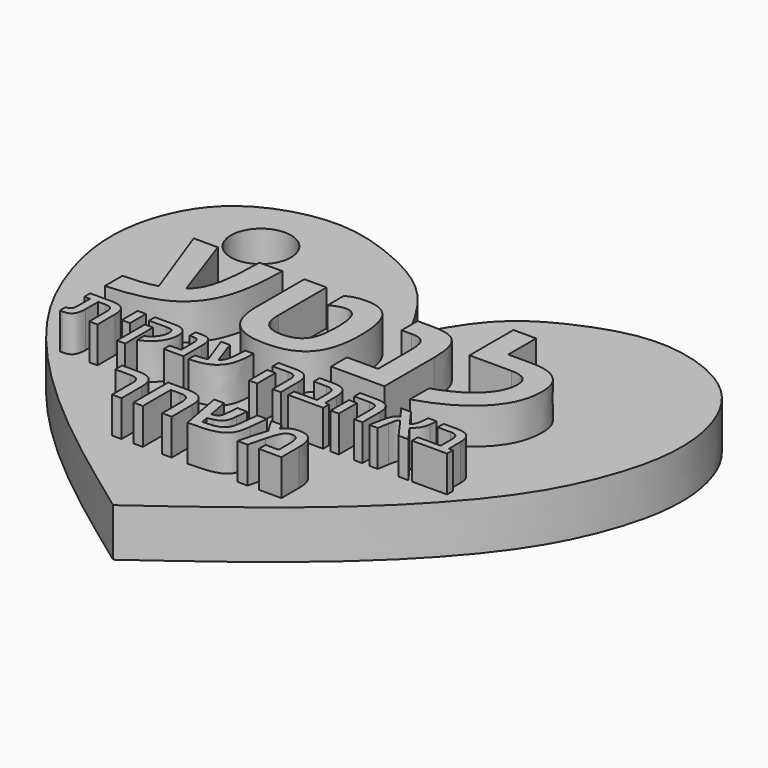
from build123d import *

# Parameters (mm, degrees)
F0_R           = 2.5
F1_DEPTH       = 4
F2_TEXT_SIZE   = 14.0530625626
F2_TEXT_SIZE_2 = 5.158657875
F2_TEXT_SIZE_3 = 5.963041874
F3_DEPTH       = 3


# Not quite as in the source:
# - Text() gives the source's letters only with a copy of the font that has no kerning and outlines rounded to 1/6400 em; it was checked with that copy


with BuildPart() as f1:
    # F0 (on Top) → F1 (new body)
    with BuildSketch(Plane.XY):
        with BuildLine():
            add(Edge.make_bspline(
                [(0, 5.3673270297), (1.0032991044, 7.2393540908), (2.9764144717, 10.9419577985), (8.4632974418, 13.8018463575), (14.0117512611, 15.2986169526), (21.7279250343, 12.71718942), (24.424666159, 4.9653958185), (22.8768308197, -1.7442714777), (20.2212687569, -7.2813165065), (15.2654507926, -13.1843862096), (8.641162767, -19.0683200173), (2.9548744589, -23.2059002096), (0, -25.355810048)],
                knots=[0, 0, 0, 0, 0.0929877273, 0.1835088349, 0.2723188941, 0.373254682, 0.4753482532, 0.5719973044, 0.6637325277, 0.7661410104, 0.8775378128, 1, 1, 1, 1], degree=3))
            add(Edge.make_bspline(
                [(0, 5.3673270297), (-1.0032991044, 7.2393540908), (-2.9764144717, 10.9419577985), (-8.4632974418, 13.8018463575), (-14.0117512611, 15.2986169526), (-21.7279250343, 12.71718942), (-24.424666159, 4.9653958185), (-22.8768308197, -1.7442714777), (-20.2212687569, -7.2813165065), (-15.2654507926, -13.1843862096), (-8.641162767, -19.0683200173), (-2.9548744589, -23.2059002096), (0, -25.355810048)],
                knots=[0, 0, 0, 0, 0.0929877273, 0.1835088349, 0.2723188941, 0.373254682, 0.4753482532, 0.5719973044, 0.6637325277, 0.7661410104, 0.8775378128, 1, 1, 1, 1], degree=3))
        make_face()
        with Locations((-15.255715698, 9.0984059498)):
            Circle(F0_R, mode=Mode.SUBTRACT)
    extrude(amount=F1_DEPTH)

    # F2 (on face) → F3 (join)
    with BuildSketch(Plane.XY.offset(4)):
        with Locations((-16.375111572, -5.7709861909)):
            Text('עטנל', F2_TEXT_SIZE, font='Arimo', font_style=FontStyle.BOLD, text_align=(TextAlign.LEFT, TextAlign.BOTTOM))
        with Locations((-16.375111572, -10.6278888683)):
            Text('תיקנע הבהאב', F2_TEXT_SIZE_2, font='Arimo', font_style=FontStyle.BOLD, text_align=(TextAlign.LEFT, TextAlign.BOTTOM))
        with Locations((-8.3389413707, -17.7498160853)):
            Text('רחשמ', F2_TEXT_SIZE_3, font='Arimo', font_style=FontStyle.BOLD, text_align=(TextAlign.LEFT, TextAlign.BOTTOM))
    extrude(amount=F3_DEPTH)


solid = f1.part
